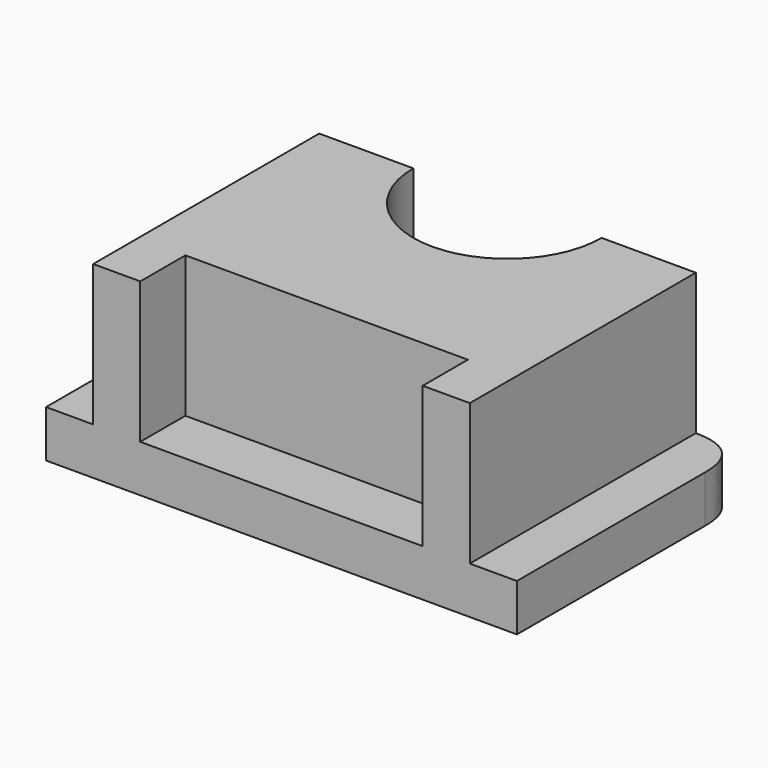
from build123d import *

# Parameters (mm, degrees)
F0_W        = 63.5
F0_H        = 38.1
F1_DEPTH    = 6.35
F2_T1_DEPTH = 38.1
F3_W        = 50.8
F3_H        = 38.1
F4_DEPTH    = 19.05
F5_W        = 38.1
F5_H        = 7.6055689663
F6_DEPTH    = 19.05
F7_R        = 12.7
F8_DEPTH    = 25.4


# Not quite as in the source:
# - a fillet or chamfer that OpenCascade refuses, or shapes differently, is made with other operations: its cross-section is extruded or revolved along the edge and cut away or added


with BuildPart() as f1:
    # F0 (on Top) → F1 (new body)
    with BuildSketch(Plane.XY):
        Rectangle(F0_W, F0_H)
    extrude(amount=F1_DEPTH)

    # F2: fillet of radius 6.35 on 2 edges, made by hand

    # F2_s2 → F2_t1 (cut)
    with BuildSketch(Plane.XY.offset(-15.875)):
        with BuildLine():
            add(Edge.make_bspline(
                [(-25.4, 19.05), (-31.75, 19.05), (-31.75, 12.7)],
                knots=[0, 0, 0, 1, 1, 1], degree=2, weights=[1, 1, 1]))
            Line((-31.75, 12.7), (-31.75, 19.05))
            Line((-31.75, 19.05), (-25.4, 19.05))
        make_face()
        with BuildLine():
            add(Edge.make_bspline(
                [(31.75, 12.7), (31.75, 19.05), (25.4, 19.05)],
                knots=[0, 0, 0, 1, 1, 1], degree=2, weights=[1, 1, 1]))
            Line((25.4, 19.05), (31.75, 19.05))
            Line((31.75, 19.05), (31.75, 12.7))
        make_face()
    extrude(amount=F2_T1_DEPTH, mode=Mode.SUBTRACT)

    # F3 (on face) → F4 (join)
    with BuildSketch(Plane.XY.offset(6.35)):
        Rectangle(F3_W, F3_H)
    extrude(amount=F4_DEPTH)

    # F5 (on face) → F6 (cut)
    with BuildSketch(Plane.XY.offset(25.4)):
        with Locations((0, -15.2472155169)):
            Rectangle(F5_W, F5_H)
    extrude(amount=-F6_DEPTH, mode=Mode.SUBTRACT)

    # F7 (on face) → F8 (cut)
    with BuildSketch(Plane.XY.offset(25.4)):
        with Locations((0, 19.05)):
            Circle(F7_R)
    extrude(amount=-F8_DEPTH, mode=Mode.SUBTRACT)


solid = f1.part
